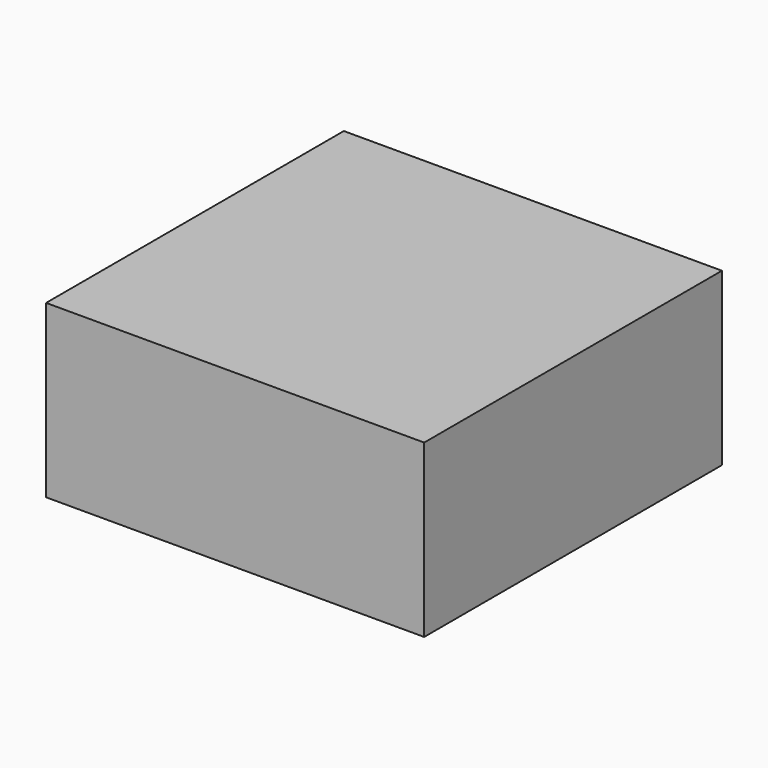
from build123d import *

# Parameters (mm, degrees)
F0_W     = 69.8630958796
F0_H     = 137.5265717506
F3_DEPTH = 63.246


# Not quite as in the source:
# - the program builds the solid bodies; features that only make, move or delete a surface that nothing else refers to are left out


with BuildPart() as f3:
    # F0 (on Top) → F3 (new body)
    with BuildSketch(Plane.XY):
        with Locations((-34.9315479398, 0)):
            Rectangle(F0_W, F0_H)
        with Locations((34.9315479398, 0)):
            Rectangle(F0_W, F0_H)
    extrude(amount=-F3_DEPTH)


solid = f3.part
